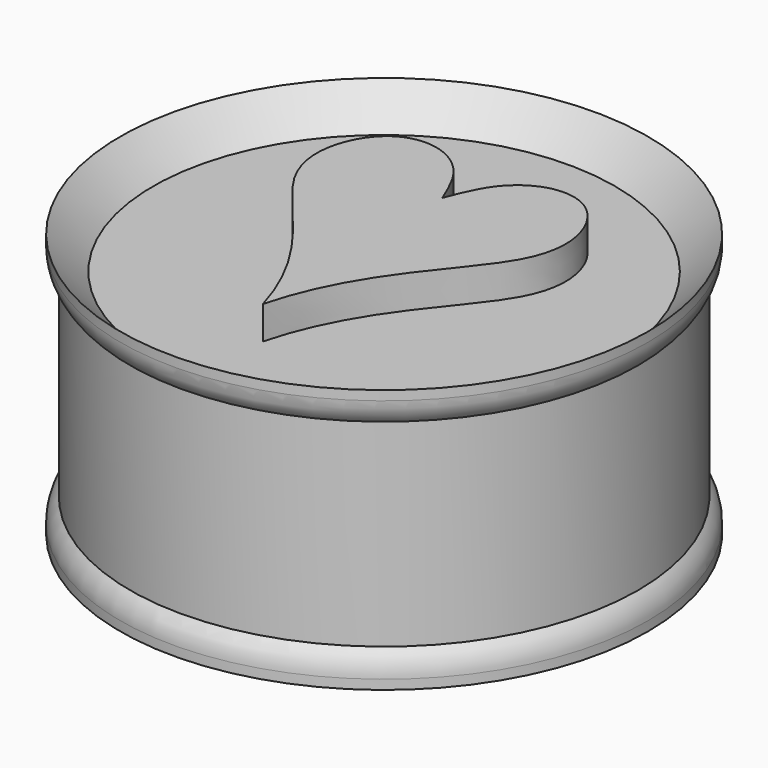
from build123d import *

# Parameters (mm, degrees)
F0_R      = 9.779
F1_DEPTH  = 7.62
F2_R      = 10.16
F2_R_2    = 8.89
F3_DEPTH  = 2.54
F5_R      = 10.16
F5_R_2    = 8.89
F6_DEPTH  = 2.54
F9_DEPTH  = 1.27
F11_DEPTH = 1.27


# Not quite as in the source:
# - a fillet or chamfer that OpenCascade refuses, or shapes differently, is made with other operations: its cross-section is extruded or revolved along the edge and cut away or added


with BuildPart() as f1:
    # F0 (on Top) → F1 (new body)
    with BuildSketch(Plane.XY):
        Circle(F0_R)
    extrude(amount=F1_DEPTH)

    # F2 (on face) → F3 (join)
    with BuildSketch(Plane.XY.offset(7.62)):
        Circle(F2_R)
        Circle(F2_R_2, mode=Mode.SUBTRACT)
    extrude(amount=F3_DEPTH)

    # F4: chamfer of 2.54 on 1 edges, made by hand


with BuildPart() as f4_tool2:
    # F4_s3 → F4_t4 (revolve)
    with BuildSketch(Plane.XZ):
        Polygon((11.43, 10.16), (8.89, 7.62), (8.89, 10.16), align=None)
    revolve(axis=Axis((0, 0, 10.16), (0, 0, 1)))

    split(bisect_by=Plane.XY.offset(7.62), keep=Keep.TOP)


with BuildPart() as f1_1:
    add(f1.part)

    # F4_t1: cut F4_tool2
    add(f4_tool2.part, mode=Mode.SUBTRACT)

    # F5 (on face) → F6 (join)
    with BuildSketch(Plane(origin=(0, 0, 0), x_dir=(1, 0, 0), z_dir=(0, 0, -1))):
        Circle(F5_R)
        Circle(F5_R_2, mode=Mode.SUBTRACT)
    extrude(amount=F6_DEPTH)

    # F7: chamfer of 2.54 on 1 edges, made by hand


with BuildPart() as f7_tool2:
    # F7_s3 → F7_t4 (revolve)
    with BuildSketch(Plane.XZ):
        Polygon((11.43, -2.54), (8.89, 0), (8.89, -2.54), align=None)
    revolve(axis=Axis((0, 0, -2.54), (0, 0, -1)))

    split(bisect_by=Plane.XY, keep=Keep.BOTTOM)


with BuildPart() as f1_2:
    add(f1_1.part)

    # F7_t1: cut F7_tool2
    add(f7_tool2.part, mode=Mode.SUBTRACT)

    # F8 (on face) → F9 (join)
    with BuildSketch(Plane.XY.offset(7.62)):
        with BuildLine():
            add(Edge.make_bspline(
                [(0, -5.8319969103), (-1.0236980804, -2.2401487669), (-4.8354001596, 0.5610413637), (-5.0054154902, 3.6583937204), (-3.9025040717, 5.331842318), (-2.2678517349, 5.574651604), (-0.814518434, 4.6455144306), (-0.3463686184, 3.5171935493), (-0.1037365128, 2.9312386094)],
                knots=[0, 0, 0, 0, 0.2996260724, 0.4641202227, 0.6025141594, 0.7280159913, 0.8588502662, 1, 1, 1, 1], degree=3))
            Line((0, -5.8319969103), (-0.1037365128, 2.9312386094))
        make_face()
        with BuildLine():
            Line((-0.1037365128, 2.9312386094), (0, -5.8319969103))
            add(Edge.make_bspline(
                [(0, -5.8319969103), (0.9383847232, -2.2169222283), (4.6827086977, 0.6737138371), (4.7793556331, 3.7742228605), (3.6371392772, 5.4210943193), (1.997197208, 5.6251399542), (0.5662657677, 4.6618597334), (0.1249568333, 3.5227729564), (-0.1037365128, 2.9312386094)],
                knots=[0, 0, 0, 0, 0.2996260724, 0.4641202227, 0.6025141594, 0.7280159913, 0.8588502662, 1, 1, 1, 1], degree=3))
        make_face()
    extrude(amount=F9_DEPTH)

    # F10 (on face) → F11 (join)
    with BuildSketch(Plane(origin=(0, 0, 0), x_dir=(1, 0, 0), z_dir=(0, 0, -1))):
        with BuildLine():
            add(Edge.make_bspline(
                [(0, 5.462912377), (1.0236980804, 1.8710642336), (4.8354001596, -0.930125897), (5.0054154902, -4.0274782537), (3.9025040717, -5.7009268513), (2.2678517349, -5.9437361373), (0.814518434, -5.0145989639), (0.3463686184, -3.8862780826), (0.1037365128, -3.3003231427)],
                knots=[0, 0, 0, 0, 0.2996260724, 0.4641202227, 0.6025141594, 0.7280159913, 0.8588502662, 1, 1, 1, 1], degree=3))
            Line((0, 5.462912377), (0.1037365128, -3.3003231427))
        make_face()
        with BuildLine():
            Line((0.1037365128, -3.3003231427), (0, 5.462912377))
            add(Edge.make_bspline(
                [(0, 5.462912377), (-0.9383847232, 1.847837695), (-4.6827086977, -1.0427983704), (-4.7793556331, -4.1433073938), (-3.6371392772, -5.7901788526), (-1.997197208, -5.9942244875), (-0.5662657677, -5.0309442667), (-0.1249568333, -3.8918574898), (0.1037365128, -3.3003231427)],
                knots=[0, 0, 0, 0, 0.2996260724, 0.4641202227, 0.6025141594, 0.7280159913, 0.8588502662, 1, 1, 1, 1], degree=3))
        make_face()
    extrude(amount=F11_DEPTH)

    # F12: fillet of radius 1.27 on 2 edges, made by hand

    # F12_s1 → F12_t2 (revolve, cut)
    with BuildSketch(Plane.XZ):
        with BuildLine():
            ThreePointArc((9.779, 0), (10.0608821461, -0.4150925255), (10.16, -0.9069614104))
            Line((10.16, -0.9069614104), (10.16, 0))
            Line((10.16, 0), (9.779, 0))
        make_face()
    revolve(axis=Axis((0, 0, 0), (0, 0, -1)), mode=Mode.SUBTRACT)

    # F12_s3 → F12_t4 (revolve, cut)
    with BuildSketch(Plane.XZ):
        with BuildLine():
            ThreePointArc((9.779, 7.62), (10.0608821461, 8.0350925255), (10.16, 8.5269614104))
            Line((10.16, 8.5269614104), (10.16, 7.62))
            Line((10.16, 7.62), (9.779, 7.62))
        make_face()
    revolve(axis=Axis((0, 0, 7.62), (0, 0, 1)), mode=Mode.SUBTRACT)


solid = f1_2.part
